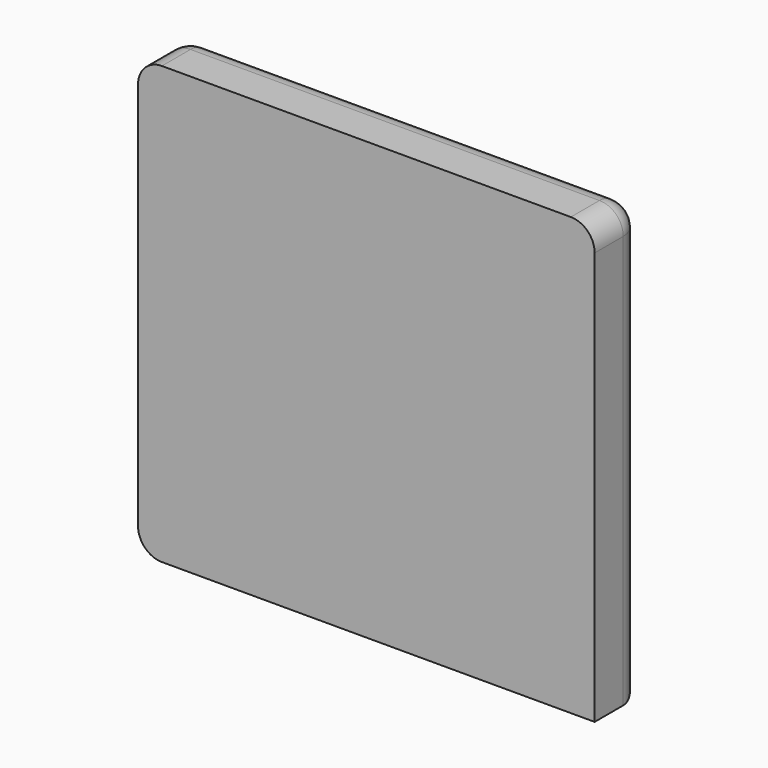
from build123d import *

# Parameters (mm, degrees)
F0_W         = 146.05
F0_H         = 139.7
F1_DEPTH     = 19.05
F2_R         = 7.62
F3_T1_DEPTH  = 30.48
F3_S5_W      = 7.62
F3_S5_H      = 7.62
F3_T6_DEPTH  = 7.62
F3_S11_W     = 7.62
F3_S11_H     = 7.62
F3_T12_DEPTH = 7.62
F4_T1_DEPTH  = 30.48
F4_S5_W      = 7.62
F4_S5_H      = 7.62
F4_T6_DEPTH  = 7.62


# Not quite as in the source:
# - a fillet or chamfer that OpenCascade refuses, or shapes differently, is made with other operations: its cross-section is extruded or revolved along the edge and cut away or added


with BuildPart() as f1:
    # F0 (on Front) → F1 (new body)
    with BuildSketch(Plane.XZ):
        Rectangle(F0_W, F0_H)
    extrude(amount=F1_DEPTH)

    # F2
    f2_edges = [f1.edges().sort_by_distance(p)[0] for p in [
        (73.025, 0, 0),
        (0, 0, 69.85),
        (-73.025, 0, 0),
        (0, 0, -69.85),
    ]]
    fillet(f2_edges, radius=F2_R)

    # F3: fillet of radius 7.62 on 2 edges, made by hand

    # F3_s2 → F3_t1 (cut)
    with BuildSketch(Plane.XZ.offset(7.62)):
        with BuildLine():
            ThreePointArc((-73.025, 62.23), (-70.7931536726, 67.6181536726), (-65.405, 69.85))
            Line((-65.405, 69.85), (-73.025, 69.85))
            Line((-73.025, 69.85), (-73.025, 62.23))
        make_face()
        with BuildLine():
            ThreePointArc((73.025, 62.23), (70.7931536726, 67.6181536726), (65.405, 69.85))
            Line((65.405, 69.85), (73.025, 69.85))
            Line((73.025, 69.85), (73.025, 62.23))
        make_face()
    extrude(amount=F3_T1_DEPTH, mode=Mode.SUBTRACT)


with BuildPart() as f3_tool4:
    # F3_s5 → F3_t6 (new body)
    with BuildSketch(Plane.YZ.offset(65.405)):
        with Locations((-3.81, 66.04)):
            Rectangle(F3_S5_W, F3_S5_H)
    extrude(amount=F3_T6_DEPTH)

    # F3_s7 → F3_t8 (revolve, cut)
    with BuildSketch(Plane(origin=(65.405, -7.62, 62.23), x_dir=(0, -0.7071067812, -0.7071067812), z_dir=(0, -0.7071067812, 0.7071067812))):
        with BuildLine():
            ThreePointArc((0, -7.62), (7.62, 0), (0, 7.62))
            Line((0, 7.62), (0, -7.62))
        make_face()
    revolve(axis=Axis((65.405, -7.62, 62.23), (1, 0, 0)), mode=Mode.SUBTRACT)


with BuildPart() as f1_1:
    add(f1.part)

    # F3_t3: cut F3_tool4
    add(f3_tool4.part, mode=Mode.SUBTRACT)


with BuildPart() as f3_tool10:
    # F3_s11 → F3_t12 (new body)
    with BuildSketch(Plane.YZ.offset(-65.405)):
        with Locations((-3.81, 66.04)):
            Rectangle(F3_S11_W, F3_S11_H)
    extrude(amount=-F3_T12_DEPTH)

    # F3_s13 → F3_t14 (revolve, cut)
    with BuildSketch(Plane(origin=(-65.405, -7.62, 62.23), x_dir=(0, -0.7071067812, -0.7071067812), z_dir=(0, 0.7071067812, -0.7071067812))):
        with BuildLine():
            ThreePointArc((0, -7.62), (7.62, 0), (0, 7.62))
            Line((0, 7.62), (0, -7.62))
        make_face()
    revolve(axis=Axis((-65.405, -7.62, 62.23), (-1, 0, 0)), mode=Mode.SUBTRACT)


with BuildPart() as f1_2:
    add(f1_1.part)

    # F3_t9: cut F3_tool10
    add(f3_tool10.part, mode=Mode.SUBTRACT)

    # F4: fillet of radius 7.62 on 1 edges, made by hand

    # F4_s2 → F4_t1 (cut)
    with BuildSketch(Plane.XZ.offset(7.62)):
        with BuildLine():
            ThreePointArc((-65.405, -69.85), (-70.7931536726, -67.6181536726), (-73.025, -62.23))
            Line((-73.025, -62.23), (-73.025, -69.85))
            Line((-73.025, -69.85), (-65.405, -69.85))
        make_face()
    extrude(amount=F4_T1_DEPTH, mode=Mode.SUBTRACT)


with BuildPart() as f4_tool4:
    # F4_s5 → F4_t6 (new body)
    with BuildSketch(Plane.XY.offset(-62.23)):
        with Locations((-69.215, -3.81)):
            Rectangle(F4_S5_W, F4_S5_H)
    extrude(amount=-F4_T6_DEPTH)

    # F4_s7 → F4_t8 (revolve, cut)
    with BuildSketch(Plane(origin=(-65.405, -7.62, -62.23), x_dir=(0.7071067812, -0.7071067812, 0), z_dir=(0.7071067812, 0.7071067812, 0))):
        with BuildLine():
            ThreePointArc((0, -7.62), (7.62, 0), (0, 7.62))
            Line((0, 7.62), (0, -7.62))
        make_face()
    revolve(axis=Axis((-65.405, -7.62, -62.23), (0, 0, -1)), mode=Mode.SUBTRACT)


with BuildPart() as f1_3:
    add(f1_2.part)

    # F4_t3: cut F4_tool4
    add(f4_tool4.part, mode=Mode.SUBTRACT)


solid = f1_3.part
